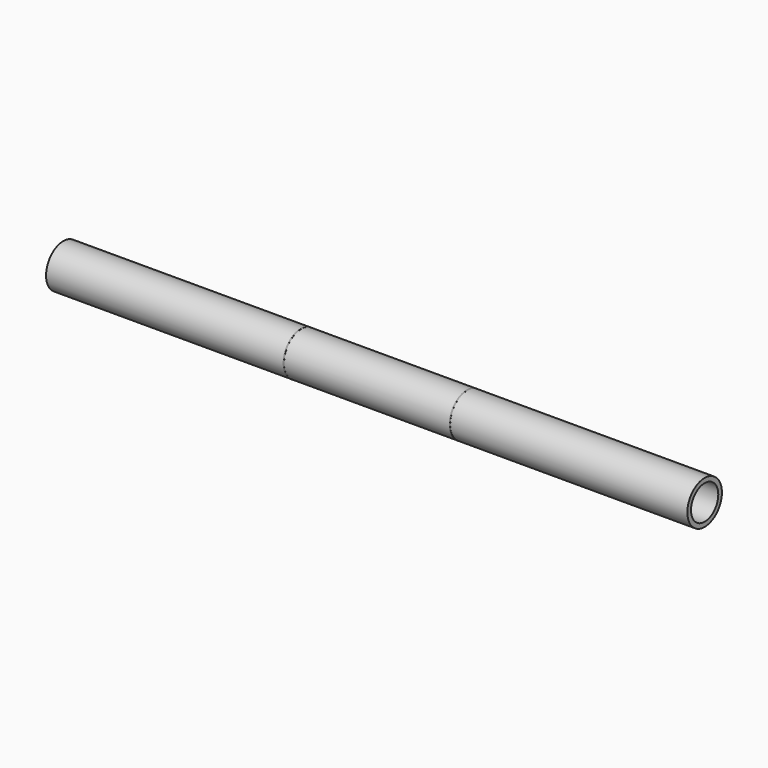
from build123d import *

# Parameters (mm, degrees)
F0_R     = 330.2
F1_DEPTH = 4902.2
F2_R     = 260.35
F3_DEPTH = 5080
F5_R     = 331.47
F6_DEPTH = 6.35


# Not quite as in the source:
# - a pattern or mirror of a feature is missing from the dataset's text; its kind, count and spacing are read off the source's solid


with BuildPart() as f1:
    # F0 (on Right) → F1 (new body, symmetric)
    with BuildSketch(Plane.YZ):
        Circle(F0_R)
    extrude(amount=F1_DEPTH, both=True)

    # F2 (on Right) → F3 (cut, symmetric)
    with BuildSketch(Plane.YZ):
        Circle(F2_R)
    extrude(amount=F3_DEPTH, both=True, mode=Mode.SUBTRACT)

    # F5 (on offset) → F6 (join, symmetric)
    with BuildSketch(Plane.YZ.offset(1270)):
        Circle(F5_R)
    f6 = extrude(amount=F6_DEPTH, both=True)

    # F6_copies: F6 across plane
    add(f6.mirror(Plane(origin=(0, 0, 0), x_dir=(0, 0, -1), z_dir=(-1, 0, 0))))


solid = f1.part
